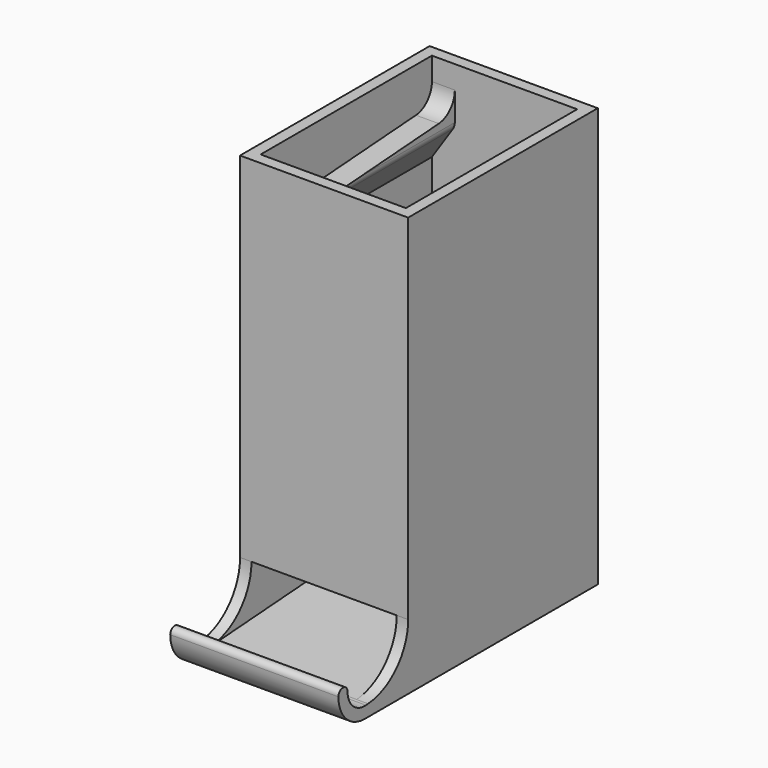
from build123d import *

# Parameters (mm, degrees)
F1_DEPTH  = 4
F2_DEPTH  = 8
F4_DEPTH  = 59.8075599705
F6_DEPTH  = 59.8075599705
F8_DEPTH  = 59.8075599705
F10_DEPTH = 59.8075599705
F11_F1_R  = 4
F11_F2_R  = 4
F11_F3_R  = 4
F11_F4_R  = 4
F11_F5_R  = 4
F11_F6_R  = 4
F11_F7_R  = 4
F11_F8_R  = 4
F14_DEPTH = 50.75
F15_R     = 7.5


with BuildPart() as f1:
    # F0 (on Right) → F1 (new body)
    with BuildSketch(Plane.YZ):
        Polygon((34.4781084829, 146.4990389768), (30.4781084829, 146.4990389768), (30.4781084829, 22.8514976037), (34.4781084829, 23.1312048515), (34.4781084829, 24.8072521052), (34.4781084829, 40.989404104), (34.4781084829, 85.147008687), (34.4781084829, 101.3291606859), align=None)
        Polygon((109.2856684534, 146.4990389768), (34.4781084829, 146.4990389768), (34.4781084829, 101.3291606859), (94.2856684534, 97.147008687), (94.2856684534, 85.147008687), (34.4781084829, 85.147008687), (34.4781084829, 40.989404104), (94.2856684534, 36.8072521052), (94.2856684534, 24.8072521052), (34.4781084829, 24.8072521052), (34.4781084829, 23.1312048515), (30.4781084829, 22.8514976037), (30.4781084829, 5.3087643873), (109.2856684534, 10.8195258131), (109.2856684534, 54.9771303961), (49.4781084829, 54.9771303961), (49.4781084829, 66.9771303961), (109.2856684534, 71.159282395), (109.2856684534, 115.3168869779), (49.4781084829, 115.3168869779), (49.4781084829, 127.3168869779), (109.2856684534, 131.4990389768), align=None)
        Polygon((109.2856684534, 115.3168869779), (109.2856684534, 131.4990389768), (49.4781084829, 127.3168869779), (49.4781084829, 115.3168869779), align=None)
        Polygon((94.2856684534, 97.147008687), (34.4781084829, 101.3291606859), (34.4781084829, 85.147008687), (94.2856684534, 85.147008687), align=None)
        Polygon((49.4781084829, 54.9771303961), (109.2856684534, 54.9771303961), (109.2856684534, 71.159282395), (49.4781084829, 66.9771303961), align=None)
        Polygon((34.4781084829, 40.989404104), (34.4781084829, 24.8072521052), (94.2856684534, 24.8072521052), (94.2856684534, 36.8072521052), align=None)
        Polygon((113.2856684534, 146.4990389768), (109.2856684534, 146.4990389768), (109.2856684534, 131.4990389768), (109.2856684534, 115.3168869779), (109.2856684534, 71.159282395), (109.2856684534, 54.9771303961), (109.2856684534, 10.8195258131), (30.4781084829, 5.3087643873), (30.4781084829, 0), (113.2856684534, 0), align=None)
        with BuildLine():
            Line((30.4781084829, 0), (30.4781084829, 5.3087643873))
            Line((30.4781084829, 5.3087643873), (12.9781084829, 4.0850451783))
            Line((12.9781084829, 4.0850451783), (12.0231735531, 4.0182696231))
            ThreePointArc((12.0231735531, 4.0182696231), (6.3850122995, 6.0148472379), (4, 11.5))
            ThreePointArc((4, 11.5), (2, 13.5), (0, 11.5))
            ThreePointArc((0, 11.5), (3.3682720164, 3.3682720164), (11.5, 0))
            Line((11.5, 0), (30.4781084829, 0))
        make_face()
        with BuildLine():
            Line((30.4781084829, 5.3087643873), (30.4781084829, 22.8514976037))
            ThreePointArc((30.4781084829, 22.8514976037), (25.4242595831, 10.0215547294), (12.9781084829, 4.0850451783))
            Line((12.9781084829, 4.0850451783), (30.4781084829, 5.3087643873))
        make_face()
    extrude(amount=-F1_DEPTH)

    # F0 (on Right) → F2 (join)
    with BuildSketch(Plane.YZ):
        Polygon((109.2856684534, 115.3168869779), (109.2856684534, 131.4990389768), (49.4781084829, 127.3168869779), (49.4781084829, 115.3168869779), align=None)
        Polygon((94.2856684534, 97.147008687), (34.4781084829, 101.3291606859), (34.4781084829, 85.147008687), (94.2856684534, 85.147008687), align=None)
        Polygon((49.4781084829, 54.9771303961), (109.2856684534, 54.9771303961), (109.2856684534, 71.159282395), (49.4781084829, 66.9771303961), align=None)
        Polygon((34.4781084829, 40.989404104), (34.4781084829, 24.8072521052), (94.2856684534, 24.8072521052), (94.2856684534, 36.8072521052), align=None)
    extrude(amount=F2_DEPTH)

    # F3 (on face) → F4 (cut, through all)
    with BuildSketch(Plane.XZ.offset(-49.4781084829)):
        Polygon((0, 115.3168869779), (8, 115.3168869779), (8, 127.3168869779), align=None)
    extrude(amount=-F4_DEPTH, mode=Mode.SUBTRACT)

    # F5 (on face) → F6 (cut, through all)
    with BuildSketch(Plane(origin=(0, 94.2856684534, 0), x_dir=(-1, 0, 0), z_dir=(0, 1, 0))):
        Polygon((-8, 85.147008687), (0, 85.147008687), (-8, 97.147008687), align=None)
    extrude(amount=-F6_DEPTH, mode=Mode.SUBTRACT)

    # F7 (on face) → F8 (cut, through all)
    with BuildSketch(Plane.XZ.offset(-49.4781084829)):
        Polygon((8, 66.9771303961), (0, 54.9771303961), (8, 54.9771303961), align=None)
    extrude(amount=-F8_DEPTH, mode=Mode.SUBTRACT)

    # F9 (on face) → F10 (cut, through all)
    with BuildSketch(Plane(origin=(0, 94.2856684534, 0), x_dir=(-1, 0, 0), z_dir=(0, 1, 0))):
        Polygon((0, 24.8072521052), (-8, 36.8072521052), (-8, 24.8072521052), align=None)
    extrude(amount=-F10_DEPTH, mode=Mode.SUBTRACT)

    # F11: fillet of radius 4 on 8 edges, made by hand

    # F11_f1
    f11_f1_edges = [f1.edges().sort_by_distance(p)[0] for p in [
        (4, 94.2856684534, 36.8072521052),
    ]]
    fillet(f11_f1_edges, radius=F11_F1_R)

    # F11_f2
    f11_f2_edges = [f1.edges().sort_by_distance(p)[0] for p in [
        (8, 63.1041505096, 36.8072521052),
    ]]
    fillet(f11_f2_edges, radius=F11_F2_R)

    # F11_f3
    f11_f3_edges = [f1.edges().sort_by_distance(p)[0] for p in [
        (4, 49.4781084829, 66.9771303961),
    ]]
    fillet(f11_f3_edges, radius=F11_F3_R)

    # F11_f4
    f11_f4_edges = [f1.edges().sort_by_distance(p)[0] for p in [
        (8, 80.6596264267, 66.9771303961),
    ]]
    fillet(f11_f4_edges, radius=F11_F4_R)

    # F11_f5
    f11_f5_edges = [f1.edges().sort_by_distance(p)[0] for p in [
        (4, 94.2856684534, 97.147008687),
    ]]
    fillet(f11_f5_edges, radius=F11_F5_R)

    # F11_f6
    f11_f6_edges = [f1.edges().sort_by_distance(p)[0] for p in [
        (8, 63.1041505096, 97.147008687),
    ]]
    fillet(f11_f6_edges, radius=F11_F6_R)

    # F11_f7
    f11_f7_edges = [f1.edges().sort_by_distance(p)[0] for p in [
        (4, 49.4781084829, 127.3168869779),
    ]]
    fillet(f11_f7_edges, radius=F11_F7_R)

    # F11_f8
    f11_f8_edges = [f1.edges().sort_by_distance(p)[0] for p in [
        (8, 80.6596264267, 127.3168869779),
    ]]
    fillet(f11_f8_edges, radius=F11_F8_R)


with BuildPart() as f12_1:
    # F12: instance of F1
    add(f1.part.mirror(Plane(origin=(0, 70.5723781379, 70.1443425212), x_dir=(0, 1, 0), z_dir=(1, 0, 0))))


with BuildPart() as f12_1_1:
    # F13: moved
    add(f12_1.part.moved(Location((50.75, 0, 0))))


with BuildPart() as f1_1:
    add(f1.part)

    add(f12_1_1.part)  # F14 merges F12_1
    # F0 (on Right) → F14 (join, through all)
    with BuildSketch(Plane.YZ):
        Polygon((34.4781084829, 146.4990389768), (30.4781084829, 146.4990389768), (30.4781084829, 22.8514976037), (34.4781084829, 23.1312048515), (34.4781084829, 24.8072521052), (34.4781084829, 40.989404104), (34.4781084829, 85.147008687), (34.4781084829, 101.3291606859), align=None)
        Polygon((113.2856684534, 146.4990389768), (109.2856684534, 146.4990389768), (109.2856684534, 131.4990389768), (109.2856684534, 115.3168869779), (109.2856684534, 71.159282395), (109.2856684534, 54.9771303961), (109.2856684534, 10.8195258131), (30.4781084829, 5.3087643873), (30.4781084829, 0), (113.2856684534, 0), align=None)
        with BuildLine():
            Line((30.4781084829, 0), (30.4781084829, 5.3087643873))
            Line((30.4781084829, 5.3087643873), (12.9781084829, 4.0850451783))
            Line((12.9781084829, 4.0850451783), (12.0231735531, 4.0182696231))
            ThreePointArc((12.0231735531, 4.0182696231), (6.3850122995, 6.0148472379), (4, 11.5))
            ThreePointArc((4, 11.5), (2, 13.5), (0, 11.5))
            ThreePointArc((0, 11.5), (3.3682720164, 3.3682720164), (11.5, 0))
            Line((11.5, 0), (30.4781084829, 0))
        make_face()
    extrude(amount=F14_DEPTH)

    # F15
    f15_edges = [f1_1.edges().sort_by_distance(p)[0] for p in [
        (4, 109.285668, 131.499039),
        (4, 109.285668, 71.159282),
        (46.75, 109.285668, 71.159282),
        (46.75, 109.285668, 131.499039),
        (4, 34.478108, 40.989404),
        (4, 34.478108, 101.329161),
        (46.75, 34.478108, 40.989404),
        (46.75, 34.478108, 101.329161),
        (25.375, 109.285668, 10.819526),
    ]]
    fillet(f15_edges, radius=F15_R)


solid = f1_1.part
